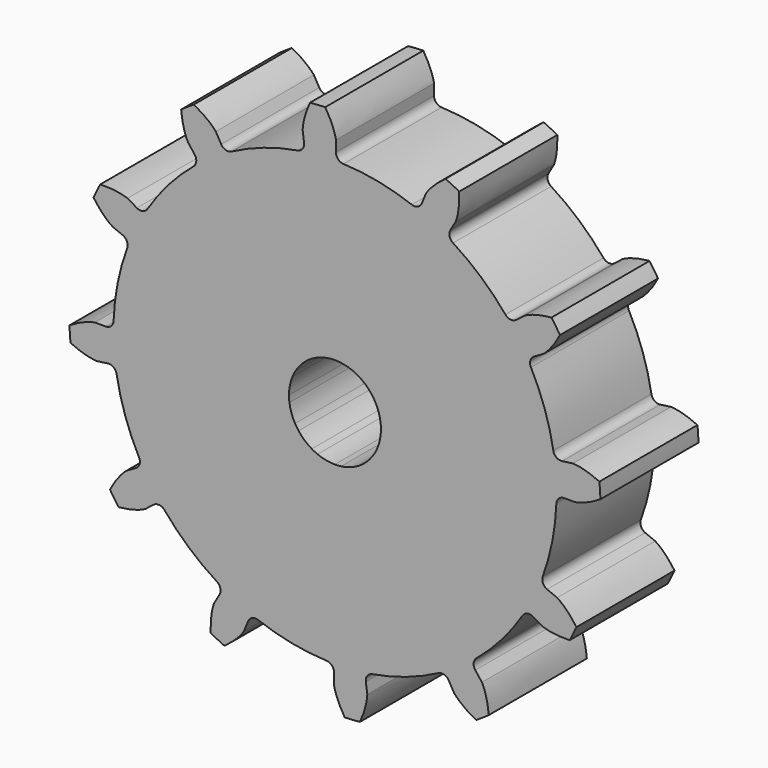
from build123d import *

# Parameters (mm, degrees)
F3_DEPTH        = 3.175
F3_COPIES_COUNT = 12
F4_R            = 0.2032


# Not quite as in the source:
# - a feature of the source that left no trace in its solid (it failed there, or was rolled back) is left out
# - a pattern or mirror of a feature is missing from the dataset's text; its kind, count and spacing are read off the source's solid


with BuildPart() as f3:
    # F2 (on Front) → F3 (new body)
    with BuildSketch(Plane.XZ):
        with BuildLine():
            add(Edge.make_bspline(
                [(-0.2524371621, 6.8745334029), (-0.1760117025, 6.7463508628), (-0.1970478939, 6.7856011476), (-0.10836209, 6.6201271318), (-0.0665643423, 6.5244260564), (-0.0277755191, 6.4234218843), (-0.0034771376, 6.349376283), (0.0198168742, 6.2543791321), (0.0153243467, 6.2727004638), (0.0260892704, 6.2183997081)],
                knots=[0, 0, 0, 0, 0.1745908743, 0.3398671109, 0.4952255417, 0.639944746, 0.7731367643, 0.8936660493, 1, 1, 1, 1], degree=3))
            ThreePointArc((-0.2524371621, 6.8745334029), (-0.4499190265, 6.8644378428), (-0.6470291412, 6.8486704781))
            add(Edge.make_bspline(
                [(-0.6470291412, 6.8486704781), (-0.7060695915, 6.7116090333), (-0.6903365579, 6.7532693004), (-0.7566649493, 6.5776351174), (-0.7856136145, 6.4772970772), (-0.8108869039, 6.3720940524), (-0.825312519, 6.2955103463), (-0.8360076309, 6.1982854305), (-0.8339449513, 6.2170364131), (-0.8375301086, 6.1617951034)],
                knots=[0, 0, 0, 0, 0.1745908743, 0.3398671109, 0.4952255417, 0.639944746, 0.7731367643, 0.8936660493, 1, 1, 1, 1], degree=3))
            Line((-0.8375301086, 6.1617951034), (-0.7727871804, 5.6854747252))
            ThreePointArc((-0.7727871804, 5.6854747252), (-0.3752670773, 5.7254691946), (0.0240725121, 5.7377036688))
            Line((0.0240725121, 5.7377036688), (0.0260892704, 6.2183997081))
        make_face()
        with BuildLine():
            Line((0.0049952183, 1.1906145213), (0.0240725121, 5.7377036688))
            ThreePointArc((0.0240725121, 5.7377036688), (-0.3752670773, 5.7254691946), (-0.7727871804, 5.6854747252))
            Line((-0.7727871804, 5.6854747252), (-0.1603588634, 1.1797766422))
            ThreePointArc((-0.1603588634, 1.1797766422), (-0.0778706007, 1.1880757805), (0.0049952183, 1.1906145213))
        make_face()
        with BuildLine():
            ThreePointArc((5.7377541667, 0), (4.0657068902, 4.0486850162), (0.0240725121, 5.7377036688))
            Line((0.0240725121, 5.7377036688), (0.0049952183, 1.1906145213))
            ThreePointArc((0.0049952183, 1.1906145213), (0.8436632392, 0.8401310787), (1.190625, 0))
            ThreePointArc((1.190625, 0), (-0.7831540777, -0.896804093), (-0.1603588634, 1.1797766422))
            Line((-0.1603588634, 1.1797766422), (-0.7727871804, 5.6854747252))
            ThreePointArc((-0.7727871804, 5.6854747252), (-3.7741065176, -4.321798569), (5.7377541667, 0))
        make_face()
    extrude(amount=F3_DEPTH)

    # F3_copies: F3 ×12 about axis
    f3_copies_axis = Axis((0, 0, 0), (0, 1, 0))


with BuildPart() as f3_1:
    add(f3.part)
    for i in range(1, F3_COPIES_COUNT):
        add(f3.part.rotate(f3_copies_axis, i * 360 / F3_COPIES_COUNT))

    # F4
    f4_edges = [f3_1.edges().sort_by_distance(p)[0] for p in [
        (-0.772787, -1.5875, 5.685475),
        (-2.848004, -1.5875, 4.981033),
        (-3.511991, -1.5875, 4.537372),
        (-4.956961, -1.5875, 2.889699),
        (-5.310159, -1.5875, 2.173484),
        (-5.737704, -1.5875, 0.024073),
        (-5.685475, -1.5875, -0.772787),
        (-4.981033, -1.5875, -2.848004),
        (-4.537372, -1.5875, -3.511991),
        (-2.889699, -1.5875, -4.956961),
        (-2.173484, -1.5875, -5.310159),
        (-0.024073, -1.5875, -5.737704),
        (0.772787, -1.5875, -5.685475),
        (2.848004, -1.5875, -4.981033),
        (3.511991, -1.5875, -4.537372),
        (4.956961, -1.5875, -2.889699),
        (5.310159, -1.5875, -2.173484),
        (5.737704, -1.5875, -0.024073),
        (5.685475, -1.5875, 0.772787),
        (4.981033, -1.5875, 2.848004),
        (4.537372, -1.5875, 3.511991),
        (2.889699, -1.5875, 4.956961),
        (2.173484, -1.5875, 5.310159),
        (0.024073, -1.5875, 5.737704),
    ]]
    fillet(f4_edges, radius=F4_R)


solid = f3_1.part
